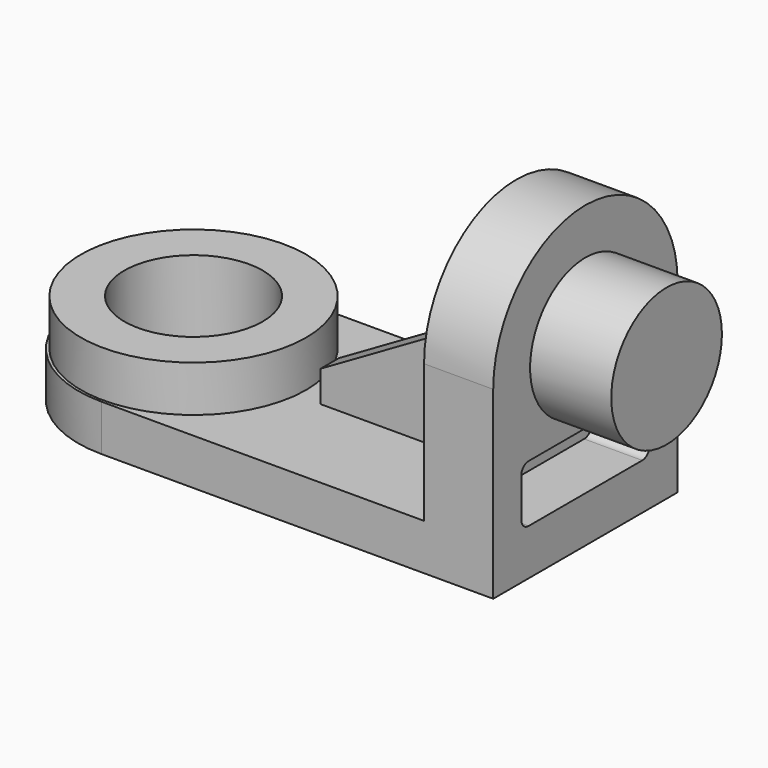
from build123d import *

# Parameters (mm, degrees)
F0_W      = 53.975
F0_H      = 31.75
F1_DEPTH  = 6.35
F2_R      = 15.5082112309
F3_DEPTH  = 6.35
F4_R      = 9.525
F5_DEPTH  = 12.7
F6_W      = 9.525
F6_H      = 19.05
F7_DEPTH  = 31.75
F9_DEPTH  = 9.525
F10_R     = 9.525
F11_DEPTH = 11.176
F13_DEPTH = 8.001
F16_DEPTH = 1.5875


# Not quite as in the source:
# - the program builds the solid bodies; features that only make, move or delete a surface that nothing else refers to are left out


with BuildPart() as f1:
    # F0 (on Top) → F1 (new body)
    with BuildSketch(Plane.XY):
        with BuildLine():
            ThreePointArc((0, 31.75), (-15.875, 15.875), (0, 0))
            Line((0, 0), (0, 31.75))
        make_face()
        with Locations((26.9875, 15.875)):
            Rectangle(F0_W, F0_H)
    extrude(amount=F1_DEPTH)

    # F2 (on face) → F3 (join)
    with BuildSketch(Plane.XY.offset(6.35)):
        with Locations((0, 15.875)):
            Circle(F2_R)
    extrude(amount=F3_DEPTH)

    # F4 (on face) → F5 (cut)
    with BuildSketch(Plane.XY.offset(12.7)):
        with Locations((0, 15.875)):
            Circle(F4_R)
    extrude(amount=-F5_DEPTH, mode=Mode.SUBTRACT)

    # F6 (on face) → F7 (join)
    with BuildSketch(Plane.XZ):
        with Locations((49.2125, 15.875)):
            Rectangle(F6_W, F6_H)
    extrude(amount=-F7_DEPTH)

    # F8 (on face) → F9 (join)
    with BuildSketch(Plane.YZ.offset(53.975)):
        with BuildLine():
            Line((0, 25.4), (31.75, 25.4))
            ThreePointArc((31.75, 25.4), (15.875, 41.275), (0, 25.4))
        make_face()
    extrude(amount=-F9_DEPTH)

    # F10 (on face) → F11 (join)
    with BuildSketch(Plane.YZ.offset(53.975)):
        with Locations((15.875, 25.4)):
            Circle(F10_R)
    extrude(amount=F11_DEPTH)

    # F12 (on face) → F13 (cut)
    with BuildSketch(Plane.YZ.offset(53.975)):
        with BuildLine():
            Line((25.654, 14.224), (6.096, 14.224))
            ThreePointArc((6.096, 14.224), (5.1979743879, 13.8520256121), (4.826, 12.954))
            Line((4.826, 12.954), (4.826, 7.62))
            ThreePointArc((4.826, 7.62), (5.1979743879, 6.7219743879), (6.096, 6.35))
            Line((6.096, 6.35), (25.654, 6.35))
            ThreePointArc((25.654, 6.35), (26.5520256121, 6.7219743879), (26.924, 7.62))
            Line((26.924, 7.62), (26.924, 12.954))
            ThreePointArc((26.924, 12.954), (26.5520256121, 13.8520256121), (25.654, 14.224))
        make_face()
    extrude(amount=-F13_DEPTH, mode=Mode.SUBTRACT)


with BuildPart() as f16:
    # F15 (on offset) → F16 (new body, symmetric)
    with BuildSketch(Plane.XZ.offset(-15.748)):
        Polygon((44.4256004055, 6.4279241487), (44.4256004055, 25.4779241487), (18.863295002, 10.719520243), (18.863295002, 6.4279241487), align=None)
    extrude(amount=F16_DEPTH, both=True)


solid = Compound([f1.part, f16.part])
